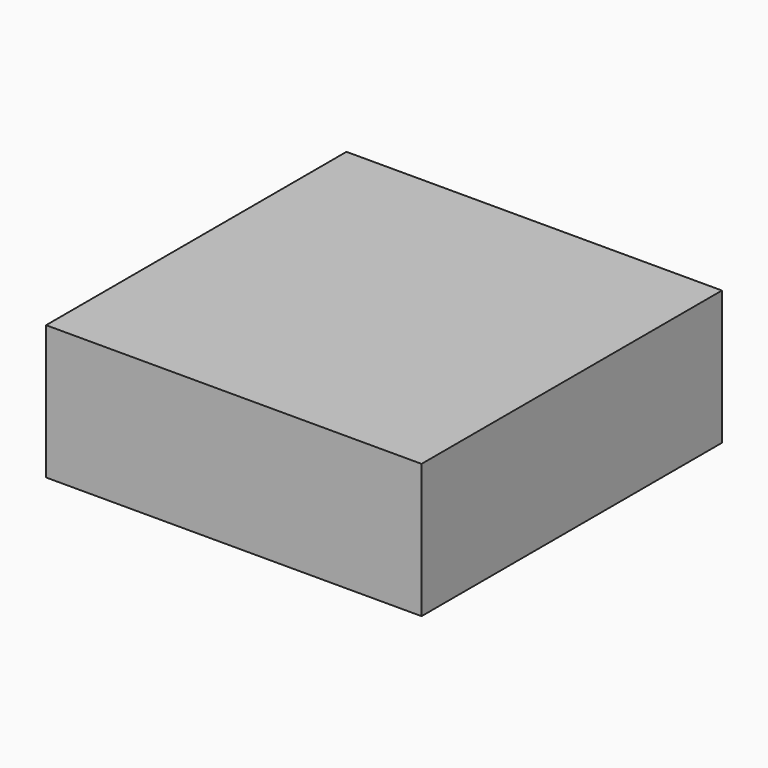
from build123d import *

# Parameters (mm, degrees)
F0_W     = 355.6
F0_H     = 355.6
F1_DEPTH = 127
F2_W     = 330.2
F2_H     = 330.2
F3_DEPTH = 114.3


# Not quite as in the source:
# - a feature names something its author has since deleted; it is built from what else it names


with BuildPart() as f1:
    # F0 (on Top) → F1 (new body)
    with BuildSketch(Plane.XY):
        Rectangle(F0_W, F0_H)
    extrude(amount=F1_DEPTH)

    # F2 (on Top) → F3 (cut)
    with BuildSketch(Plane.XY):
        Rectangle(F2_W, F2_H)
    extrude(amount=F3_DEPTH, mode=Mode.SUBTRACT)


solid = f1.part
